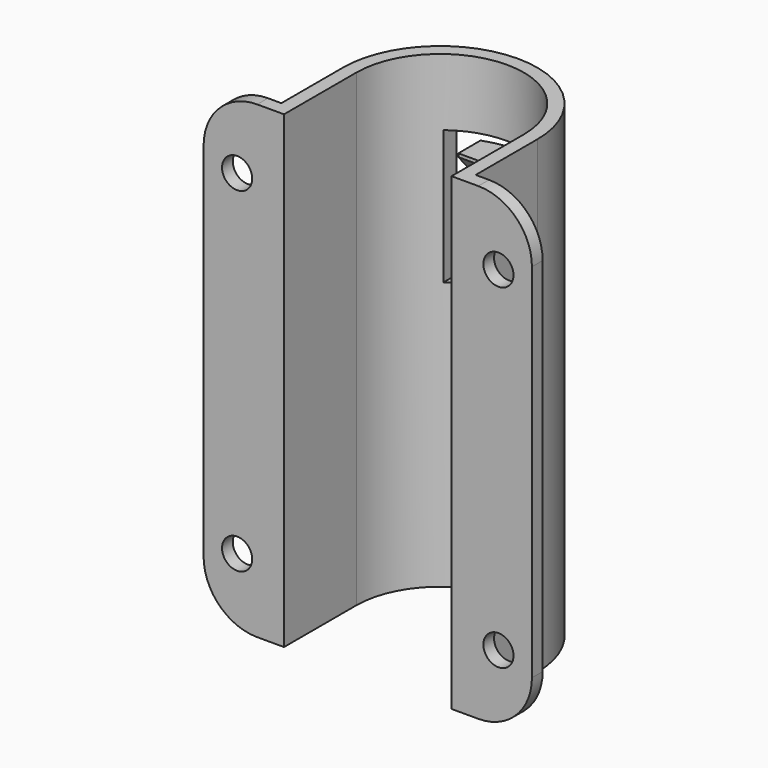
from build123d import *

# Parameters (mm, degrees)
F1_DEPTH     = 35
F3_D         = 4.5
F7_REACH     = 50.3610093633
F8_R         = 8
F10_DEPTH    = 4
F11_T4_DEPTH = 27.8083046081
F11_S5_R     = 12.5
F11_T6_DEPTH = 16


# Not quite as in the source:
# - a fillet or chamfer that OpenCascade refuses, or shapes differently, is made with other operations: its cross-section is extruded or revolved along the edge and cut away or added
# - a pattern or mirror of a feature is missing from the dataset's text; its kind, count and spacing are read off the source's solid


with BuildPart() as f1:
    # F0 (on Top) → F1 (new body, symmetric)
    with BuildSketch(Plane.XY):
        with BuildLine():
            Line((-24.5, 2), (-24.5, 0))
            Line((-24.5, 0), (-12.5, 0))
            Line((-12.5, 0), (-12.5, 13.5))
            ThreePointArc((-12.5, 13.5), (-8.8388347648, 22.3388347648), (0, 26))
            Line((0, 26), (0, 28))
            ThreePointArc((0, 28), (-10.2530483272, 23.7530483272), (-14.5, 13.5))
            Line((-14.5, 13.5), (-14.5, 2))
            Line((-14.5, 2), (-24.5, 2))
        make_face()
    extrude(amount=F1_DEPTH, both=True)

    # F3 (through all)
    with Locations(Plane(origin=(0, 2, 0), x_dir=(-1, 0, 0), z_dir=(0, 1, 0))):
        with Locations((19.5, -25), (19.5, 25)):
            Hole(F3_D / 2)

    # F4: F1 across plane


with BuildPart() as f1_1:
    add(f1.part)
    add(f1.part.mirror(Plane.YZ))

    f7_end = f1_1.faces().sort_by_distance((0, 26, 0))[0]
    # F6 (on offset) → F7 (cut, up to a face of the model that its end follows)
    with BuildSketch(Plane.XZ.offset(-29)):
        Polygon((0, 23), (0, 25), (-7.5, 25), (-7.5, 5), (-4.8855356313, 5), (-4.8855356313, 23), align=None)
    f7_long = extrude(amount=F7_REACH, mode=Mode.PRIVATE)
    f7 = split(f7_long, bisect_by=f7_end, keep=Keep.BOTTOM, mode=Mode.PRIVATE)
    add(f7, mode=Mode.SUBTRACT)

    # F7_copies: F7 across plane
    add(f7.mirror(Plane(origin=(0, 0, 0), x_dir=(0, 0, 1), z_dir=(1, 0, 0))), mode=Mode.SUBTRACT)

    # F8
    f8_edges = [f1_1.edges().sort_by_distance(p)[0] for p in [
        (-24.5, 1, -35),
        (24.5, 1, -35),
        (-24.5, 1, 35),
        (24.5, 1, 35),
    ]]
    fillet(f8_edges, radius=F8_R)

    # F9 (on face) → F10 (join)
    with BuildSketch(Plane.XY.offset(23)):
        with BuildLine():
            ThreePointArc((4.8855356313, 25.0057177783), (0, 26), (-4.8855356313, 25.0057177783))
            Line((-4.8855356313, 25.0057177783), (-4.8855356313, 23.0057177783))
            Line((-4.8855356313, 23.0057177783), (4.8855356313, 23.0057177783))
            Line((4.8855356313, 23.0057177783), (4.8855356313, 25.0057177783))
        make_face()
    extrude(amount=-F10_DEPTH)

    # F11: chamfer of 3 x 3.5 on 1 edges, made by hand


with BuildPart() as f11_tool2:
    # F11_s3 → F11_t4 (new body)
    with BuildSketch(Plane.YZ.offset(-13.9041523041)):
        Polygon((23.0057177783, 22.5), (26.0057177783, 19), (23.0057177783, 19), align=None)
    extrude(amount=F11_T4_DEPTH)

    # F11_s5 → F11_t6 (intersect, symmetric)
    with BuildSketch(Plane.XY.offset(20.8)):
        with Locations((0, 13.5)):
            Circle(F11_S5_R)
    extrude(amount=F11_T6_DEPTH, both=True, mode=Mode.INTERSECT)


with BuildPart() as f1_2:
    add(f1_1.part)

    # F11_t1: cut F11_tool2
    add(f11_tool2.part, mode=Mode.SUBTRACT)


solid = f1_2.part
